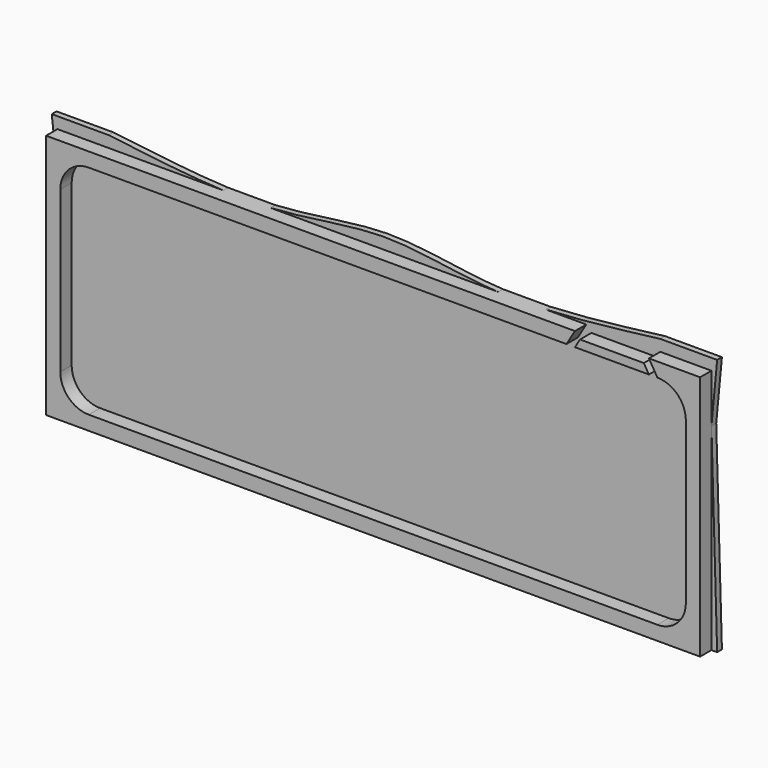
from build123d import *

# Parameters (mm, degrees)
F0_W     = 584.2
F0_H     = 219.71
F1_DEPTH = 5.334
F2_W     = 558.8
F2_H     = 194.31
F3_DEPTH = 12.7
F4_R     = 25.4
F6_DEPTH = 12.7
F8_DEPTH = 5.334


# Not quite as in the source:
# - a feature names something its author has since deleted; it is built from what else it names


with BuildPart() as f1:
    # F0 (on Front) → F1 (new body)
    with BuildSketch(Plane.XZ):
        with Locations((-292.1, 109.855)):
            Rectangle(F0_W, F0_H)
    extrude(amount=F1_DEPTH)

    # F2 (on face) → F3 (join)
    with BuildSketch(Plane.XZ.offset(5.334)):
        Polygon((0, 219.71), (-6.35, 219.71), (-577.85, 219.71), (-584.2, 219.71), (-584.2, 0), (0, 0), align=None)
        with Locations((-292.1, 109.855)):
            Rectangle(F2_W, F2_H, mode=Mode.SUBTRACT)
    extrude(amount=F3_DEPTH)

    # F4
    f4_edges = [f1.edges().sort_by_distance(p)[0] for p in [
        (-571.5, -11.684, 207.01),
        (-12.7, -11.684, 207.01),
        (-12.7, -11.684, 12.7),
        (-571.5, -11.684, 12.7),
    ]]
    fillet(f4_edges, radius=F4_R)

    # F5 (on face) → F6 (cut)
    with BuildSketch(Plane.XZ.offset(18.034)):
        Polygon((-104.14, 219.71), (-111.76, 219.71), (-119.38, 207.01), (-111.76, 207.01), (-107.2320166854, 214.5566388576), align=None)
        Polygon((-38.1, 207.01), (-45.72, 219.71), (-53.34, 219.71), (-50.2479833146, 214.5566388576), (-45.72, 207.01), align=None)
        Polygon((-53.34, 219.71), (-104.14, 219.71), (-107.2320166854, 214.5566388576), (-50.2479833146, 214.5566388576), align=None)
    extrude(amount=-F6_DEPTH, mode=Mode.SUBTRACT)

    # F7 (on face) → F8 (join)
    with BuildSketch(Plane(origin=(0, 0, 0), x_dir=(-1, 0, 0), z_dir=(0, 1, 0))):
        with BuildLine():
            Line((-5.08, 229.87), (0, 176.1275827885))
            Line((0, 176.1275827885), (0, 219.71))
            Line((0, 219.71), (148.0852009026, 219.71))
            add(Edge.make_bspline(
                [(148.0852009026, 219.71), (115.3779899576, 221.1840971885), (80.5489949788, 225.5270485943), (45.72, 229.87)],
                knots=[0.812101374, 0.812101374, 0.812101374, 0.812101374, 1, 1, 1, 1], degree=3))
            Line((45.72, 229.87), (-5.08, 229.87))
        make_face()
        with BuildLine():
            add(Edge.make_bspline(
                [(393.7, 219.71), (356.8171998762, 221.731425099), (324.4585999381, 229.87), (292.1, 229.87)],
                knots=[0.2719218593, 0.2719218593, 0.2719218593, 0.2719218593, 0.5, 0.5, 0.5, 0.5], degree=3))
            add(Edge.make_bspline(
                [(292.1, 229.87), (259.7414000619, 229.87), (227.3828001238, 221.731425099), (190.5, 219.71)],
                knots=[0.5, 0.5, 0.5, 0.5, 0.7280781407, 0.7280781407, 0.7280781407, 0.7280781407], degree=3))
            Line((190.5, 219.71), (393.7, 219.71))
        make_face()
        Polygon((584.2, 183.2547038794), (584.2, 0), (589.28, 0), align=None)
        with BuildLine():
            Line((584.2, 219.71), (584.2, 183.2547038794))
            Line((584.2, 183.2547038794), (589.28, 229.87))
            Line((589.28, 229.87), (538.48, 229.87))
            add(Edge.make_bspline(
                [(538.48, 229.87), (503.6510050212, 225.5270485943), (468.8220100424, 221.1840971885), (436.1147990974, 219.71)],
                knots=[0, 0, 0, 0, 0.187898626, 0.187898626, 0.187898626, 0.187898626], degree=3))
            Line((436.1147990974, 219.71), (584.2, 219.71))
        make_face()
        Polygon((-5.08, 0), (0, 0), (0, 176.1275827885), align=None)
    extrude(amount=-F8_DEPTH)


solid = f1.part
